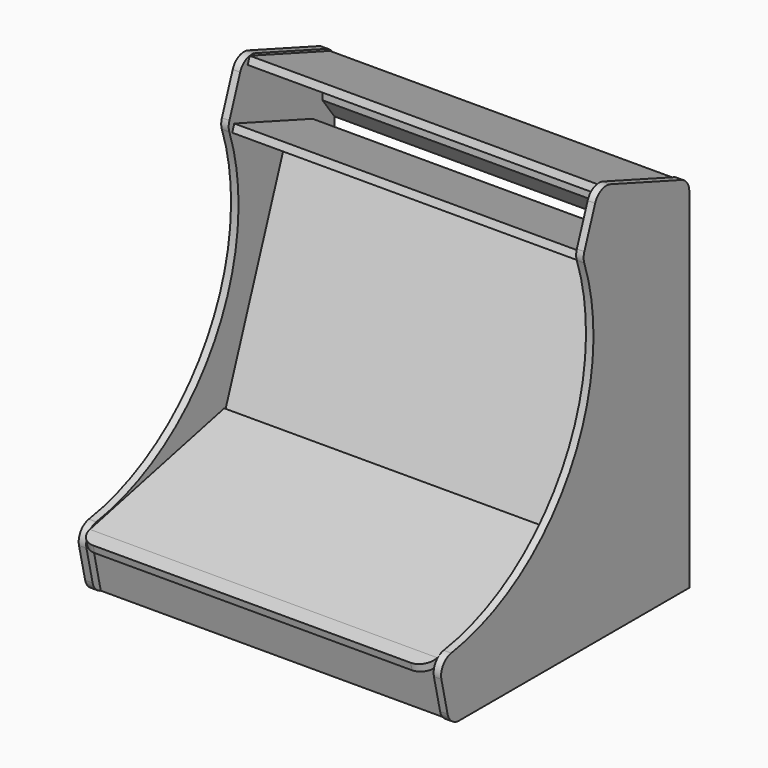
from build123d import *

# Parameters (mm, degrees)
F3_DEPTH  = 12.7
F6_DEPTH  = 12.7
F7_R      = 25.4
F7_2_R    = 25.4
F9_DEPTH  = 294.64
F10_DEPTH = 294.64
F11_DEPTH = 294.64
F12_DEPTH = 25.4
F13_R     = 25.4
F15_DEPTH = 294.64
F17_DEPTH = 294.64
F18_W     = 254
F18_H     = 12.7
F19_DEPTH = 294.64
F20_W     = 12.7
F20_H     = 152.4
F21_DEPTH = 294.64
F23_DEPTH = 293.37
F25_DEPTH = 294.64


with BuildPart() as f3:
    # F2 (on offset) → F3 (new body)
    with BuildSketch(Plane.YZ.offset(294.64)):
        with BuildLine():
            Line((-508, 0), (0, 0))
            Line((0, 0), (0, 609.6))
            Line((0, 609.6), (-190.9455405437, 679.0984931238))
            Line((-190.9455405437, 679.0984931238), (-225.6947871056, 583.6257228519))
            ThreePointArc((-225.6947871056, 583.6257228519), (-259.177173919, 267.6439817216), (-531.8944548557, 104.5770763332))
            Line((-531.8944548557, 104.5770763332), (-508, 0))
        make_face()
    extrude(amount=F3_DEPTH)

    # F7
    f7_edges = [f3.edges().sort_by_distance(p)[0] for p in [
        (300.99, 0, 609.6),
        (300.99, -190.945541, 679.098493),
        (300.99, -225.694787, 583.625723),
        (300.99, -531.894455, 104.577076),
        (300.99, -508, 0),
    ]]
    fillet(f7_edges, radius=F7_R)


with BuildPart() as f6:
    # F5 (on offset) → F6 (new body)
    with BuildSketch(Plane.YZ.offset(-294.64)):
        with BuildLine():
            Line((-508, 0), (0, 0))
            Line((0, 0), (0, 609.6))
            Line((0, 609.6), (-190.9455405437, 679.0984931238))
            Line((-190.9455405437, 679.0984931238), (-225.6947871056, 583.6257228519))
            ThreePointArc((-225.6947871056, 583.6257228519), (-259.177173919, 267.6439817216), (-531.8944548557, 104.5770763332))
            Line((-531.8944548557, 104.5770763332), (-508, 0))
        make_face()
    extrude(amount=-F6_DEPTH)

    # F7#2
    f7_2_edges = [f6.edges().sort_by_distance(p)[0] for p in [
        (-300.99, -225.694787, 583.625723),
        (-300.99, -190.945541, 679.098493),
        (-300.99, 0, 609.6),
        (-300.99, -531.894455, 104.577076),
        (-300.99, -508, 0),
    ]]
    fillet(f7_2_edges, radius=F7_2_R)


with BuildPart() as f9:
    # F8 (on Right) → F9 (new body, symmetric)
    with BuildSketch(Plane.YZ):
        Polygon((-518.2986226671, 102.0887864602), (-515.4697464551, 89.7078551795), (-503.0888151744, 92.5367313915), (-236.8987926395, 153.3575699491), (-233.5372032111, 167.1529393358), align=None)
    extrude(amount=F9_DEPTH, both=True)

    # F12 (add): a face of the model
    f12_faces = [f9.faces().sort_by_distance(p)[0] for p in [
        (0, -516.8841845611, 95.8983208198),
    ]]
    extrude(f12_faces, amount=F12_DEPTH)

    # F13
    f13_edges = [f9.edges().sort_by_distance(p)[0] for p in [
        (-294.64, -541.646047, 90.240568),
        (294.64, -541.646047, 90.240568),
    ]]
    fillet(f13_edges, radius=F13_R)


with BuildPart() as f10:
    # F8 (on Right) → F10 (new body, symmetric)
    with BuildSketch(Plane.YZ):
        Polygon((-515.4697464551, 89.7078551795), (-495.24789644, 1.204394213), (-482.6999233712, 3.3021911042), (-503.0888151744, 92.5367313915), align=None)
    extrude(amount=F10_DEPTH, both=True)


with BuildPart() as f11:
    # F0 (on Right) → F11 (new body, symmetric)
    with BuildSketch(Plane.YZ):
        Polygon((-25.4, 542.5802856922), (0, 508), (0, 558.8), (-25.4, 558.8), align=None)
    extrude(amount=F11_DEPTH, both=True)


with BuildPart() as f15:
    # F14 (on Right) → F15 (new body, symmetric)
    with BuildSketch(Plane.YZ):
        Polygon((-9.4422581348, 609.6579364777), (-179.5031301816, 671.5550319161), (-183.8467860018, 659.6209356321), (-13.7859139551, 597.7238401937), align=None)
    extrude(amount=F15_DEPTH, both=True)


with BuildPart() as f17:
    # F16 (on Right) → F17 (new body, symmetric)
    with BuildSketch(Plane.YZ):
        Polygon((-46.2742848321, 523.2568957286), (-212.1746461021, 583.6396890849), (-216.5183019223, 571.7055928009), (-50.6179406523, 511.3227994446), align=None)
    extrude(amount=F17_DEPTH, both=True)


with BuildPart() as f19:
    # F18 (on Right) → F19 (new body, symmetric)
    with BuildSketch(Plane.YZ):
        with Locations((-127, 6.35)):
            Rectangle(F18_W, F18_H)
    extrude(amount=F19_DEPTH, both=True)


with BuildPart() as f21:
    # F20 (on Right) → F21 (new body, symmetric)
    with BuildSketch(Plane.YZ):
        with Locations((-6.35, 88.9)):
            Rectangle(F20_W, F20_H)
    extrude(amount=F21_DEPTH, both=True)


with BuildPart() as f23:
    # F22 (on Right) → F23 (new body, symmetric)
    with BuildSketch(Plane.YZ):
        Polygon((-88.9741059927, 522.5294433083), (-100.9082022767, 526.8730991285), (-239.9051885242, 144.9820180411), (-227.9710922402, 140.6383622209), align=None)
    extrude(amount=F23_DEPTH, both=True)


with BuildPart() as f25:
    # F24 (on Right) → F25 (new body, symmetric)
    with BuildSketch(Plane.YZ):
        Polygon((-194.8436558202, 115.065903716), (-190.5, 127), (-239.9051885242, 144.9820180411), (-243.9318360877, 132.9325401877), align=None)
    extrude(amount=F25_DEPTH, both=True)


solid = Compound([f3.part, f6.part, f9.part, f10.part, f11.part, f15.part, f17.part, f19.part, f21.part, f23.part, f25.part])
